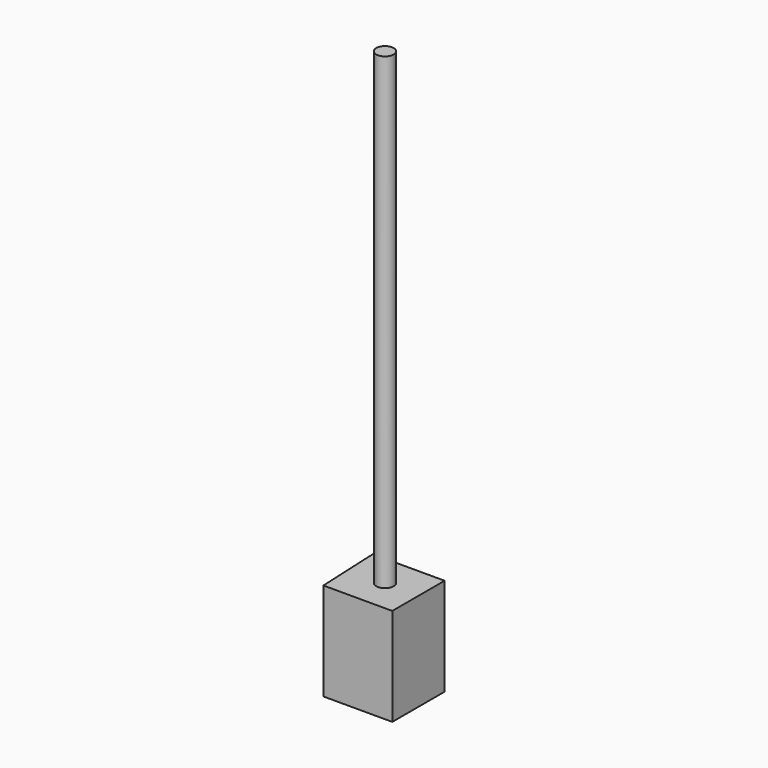
from build123d import *

# Parameters (mm, degrees)
F1_DEPTH = 84.7620591521
F2_R     = 7.5874829839
F3_DEPTH = 406.0934484005


# Not quite as in the source:
# - the program builds the solid bodies; features that only make, move or delete a surface that nothing else refers to are left out


with BuildPart() as f1:
    # F0 (on Top) → F1 (new body)
    with BuildSketch(Plane.XY):
        Polygon((29.4313300401, 27.8682895005), (-32.9063385725, 27.8682895005), (-30.3279589862, -28.8718193769), (29.4313300401, -28.8718193769), align=None)
    extrude(amount=-F1_DEPTH)

    # F2 (on Top) → F3 (join)
    with BuildSketch(Plane.XY):
        Circle(F2_R)
    extrude(amount=F3_DEPTH)


solid = f1.part
